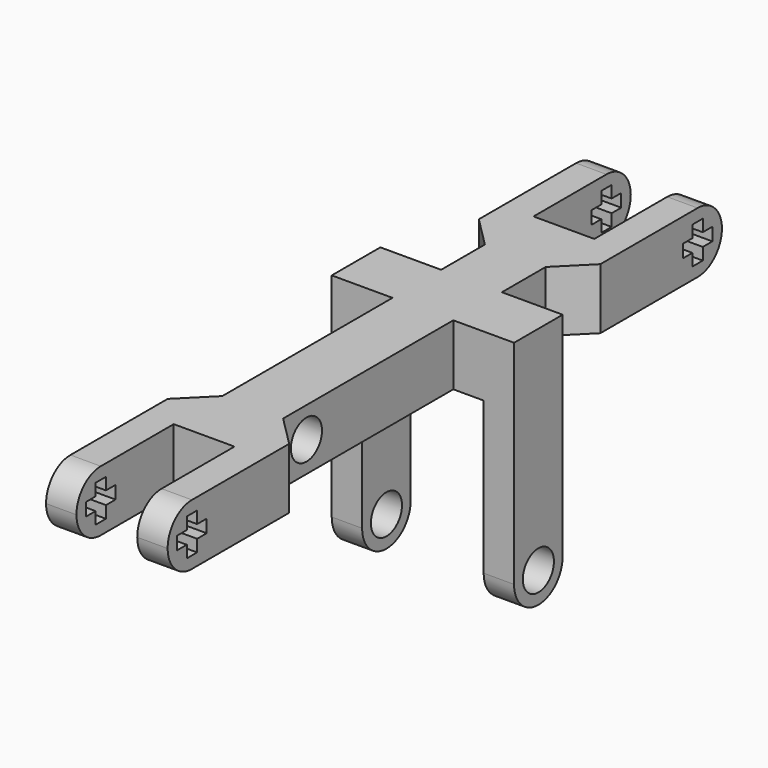
from build123d import *

# Parameters (mm, degrees)
F1_DEPTH  = 7.9375
F2_R      = 2.54
F2_W      = 1.6891
F2_H      = 1.56845
F2_H_2    = 1.6891
F2_W_2    = 1.56845
F3_DEPTH  = 15.875
F4_SIZE   = 3.96874
F5_W      = 7.9375
F5_H      = 7.9375
F6_DEPTH  = 7.9375
F7_W      = 3.96875
F7_H      = 7.9375
F8_DEPTH  = 23.8125
F9_R      = 3.96874
F10_R     = 2.54
F11_DEPTH = 23.8125
F12_W     = 1.6891
F12_H     = 1.56845
F12_W_2   = 1.56845
F12_H_2   = 1.6891
F13_DEPTH = 15.875


# Not quite as in the source:
# - a fillet or chamfer is up to 0.001 mm smaller than in the source, because OpenCascade refuses the exact size


with BuildPart() as f1:
    # F0 (on Top) → F1 (new body)
    with BuildSketch(Plane.XY):
        Polygon((3.96875, 0), (0, 0), (0, -19.84375), (3.96875, -19.84375), (3.96875, -3.96875), (11.90625, -3.96875), (11.90625, -19.84375), (15.875, -19.84375), (15.875, 0), (11.90625, 0), (11.90625, 50.8), (15.875, 50.8), (15.875, 70.64375), (11.90625, 70.64375), (11.90625, 54.76875), (3.96875, 54.76875), (3.96875, 70.64375), (0, 70.64375), (0, 50.8), (3.96875, 50.8), align=None)
    extrude(amount=F1_DEPTH)

    # F2 (on face) → F3 (cut, through all)
    with BuildSketch(Plane.YZ.offset(15.875)):
        with BuildLine():
            ThreePointArc((-15.875, 0), (-18.6813300378, 1.1624199622), (-19.84375, 3.96875))
            Line((-19.84375, 3.96875), (-19.84375, 0))
            Line((-19.84375, 0), (-15.875, 0))
        make_face()
        with BuildLine():
            ThreePointArc((-19.84375, 3.96875), (-18.6813300378, 6.7750800378), (-15.875, 7.9375))
            Line((-15.875, 7.9375), (-19.84375, 7.9375))
            Line((-19.84375, 7.9375), (-19.84375, 3.96875))
        make_face()
        with Locations((7.778559196, 3.96875)):
            Circle(F2_R)
        with Locations((-15.875, 5.597525)):
            Rectangle(F2_W, F2_H)
        with Locations((-15.875, 3.96875)):
            Rectangle(F2_W, F2_H_2)
        with Locations((-17.503775, 3.96875)):
            Rectangle(F2_W_2, F2_H_2)
        with Locations((-14.246225, 3.96875)):
            Rectangle(F2_W_2, F2_H_2)
        with Locations((-15.875, 2.339975)):
            Rectangle(F2_W, F2_H)
    extrude(amount=-F3_DEPTH, mode=Mode.SUBTRACT)

    # F4 (size 3.96875 in the source; OpenCascade refuses exactly that, so slightly less here)
    f4_edges = [f1.edges().sort_by_distance(p)[0] for p in [
        (11.90625, 0, 3.96875),
        (3.96875, 0, 3.96875),
        (11.90625, 50.8, 3.96875),
        (3.96875, 50.8, 3.96875),
    ]]
    chamfer(f4_edges, length=F4_SIZE)

    # F5 (on face) → F6 (join, through all)
    with BuildSketch(Plane.XY.offset(7.9375)):
        with Locations((0, 35.71875)):
            Rectangle(F5_W, F5_H)
        with Locations((15.875, 35.71875)):
            Rectangle(F5_W, F5_H)
    extrude(amount=-F6_DEPTH)

    # F7 (on face) → F8 (join)
    with BuildSketch(Plane(origin=(0, 0, 0), x_dir=(1, 0, 0), z_dir=(0, 0, -1))):
        with Locations((17.859375, -35.71875)):
            Rectangle(F7_W, F7_H)
        with Locations((-1.984375, -35.71875)):
            Rectangle(F7_W, F7_H)
    extrude(amount=F8_DEPTH)

    # F9 (radius 3.96875 in the source; OpenCascade refuses exactly that, so slightly less here)
    f9_edges = [f1.edges().sort_by_distance(p)[0] for p in [
        (-1.984375, 39.6875, -23.8125),
        (-1.984375, 31.75, -23.8125),
        (17.859375, 31.75, -23.8125),
        (17.859375, 39.6875, -23.8125),
        (13.890625, 70.64375, 0),
        (13.890625, 70.64375, 7.9375),
        (1.984375, 70.64375, 7.9375),
        (1.984375, 70.64375, 0),
    ]]
    fillet(f9_edges, radius=F9_R)

    # F10 (on face) → F11 (cut, through all)
    with BuildSketch(Plane(origin=(-3.96875, 0, 0), x_dir=(0, -1, 0), z_dir=(-1, 0, 0))):
        with Locations((-35.71875, -19.84375)):
            Circle(F10_R)
    extrude(amount=-F11_DEPTH, mode=Mode.SUBTRACT)

    # F12 (on face) → F13 (cut, through all)
    with BuildSketch(Plane.YZ.offset(15.875)):
        with Locations((66.675, 2.339975)):
            Rectangle(F12_W, F12_H)
        with Locations((65.046225, 3.96875)):
            Rectangle(F12_W_2, F12_H_2)
        with Locations((66.675, 3.96875)):
            Rectangle(F12_W, F12_H_2)
        with Locations((68.303775, 3.96875)):
            Rectangle(F12_W_2, F12_H_2)
        with Locations((66.675, 5.597525)):
            Rectangle(F12_W, F12_H)
    extrude(amount=-F13_DEPTH, mode=Mode.SUBTRACT)


solid = f1.part
